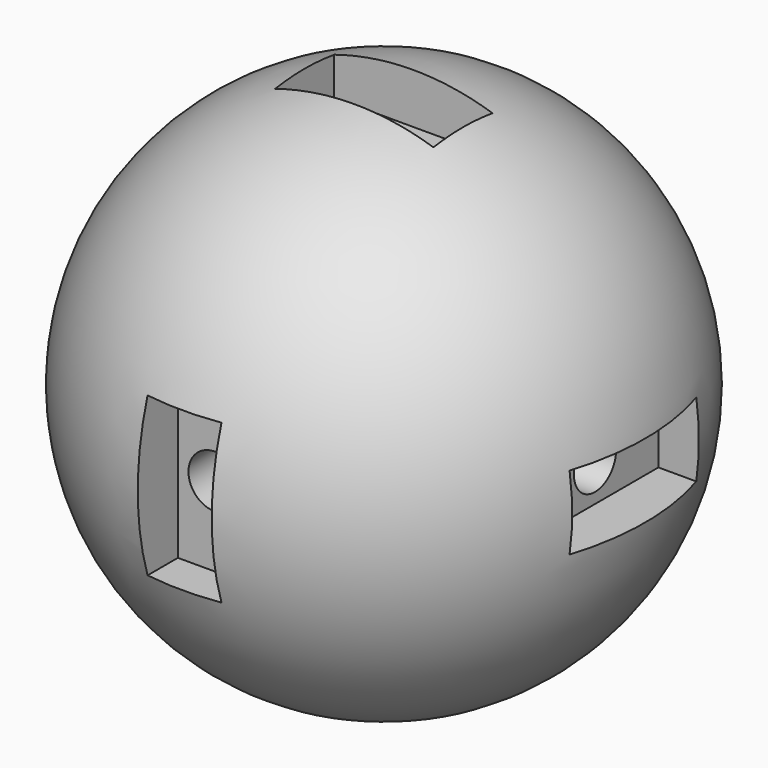
from build123d import *

# Parameters (mm, degrees)
F3_W      = 7
F3_H      = 15
F4_DEPTH  = 5
F5_R      = 2.5
F6_DEPTH  = 45.001
F8_W      = 15
F8_H      = 7
F9_DEPTH  = 5
F10_R     = 2.5
F11_DEPTH = 44.754787589
F13_W     = 15
F13_H     = 7
F14_DEPTH = 5
F15_R     = 2.5
F16_DEPTH = 44.754787589


# Not quite as in the source:
# - a pattern or mirror of a feature is missing from the dataset's text; its kind, count and spacing are read off the source's solid


with BuildPart() as f1:
    # F0 (on Front) → F1 (revolve)
    with BuildSketch(Plane.XZ):
        with BuildLine():
            Line((0, -25), (0, 25))
            ThreePointArc((0, 25), (-25, 0), (0, -25))
        make_face()
    revolve(axis=Axis((0, 0, 0), (0, 0, -1)))

    # F3 (on offset) → F4 (cut)
    with BuildSketch(Plane.XZ.offset(25)):
        Rectangle(F3_W, F3_H)
    f4 = extrude(amount=-F4_DEPTH, mode=Mode.SUBTRACT)

    # F4_copies: F4 across plane
    add(f4.mirror(Plane.ZX), mode=Mode.SUBTRACT)

    # F5 (on face) → F6 (cut, through all)
    with BuildSketch(Plane.XZ.offset(20)):
        Circle(F5_R)
    extrude(amount=-F6_DEPTH, mode=Mode.SUBTRACT)

    # F8 (on offset) → F9 (cut)
    with BuildSketch(Plane.XY.offset(25)):
        Rectangle(F8_W, F8_H)
    f9 = extrude(amount=-F9_DEPTH, mode=Mode.SUBTRACT)

    # F9_copies: F9 across plane
    add(f9.mirror(Plane(origin=(0, 0, 0), x_dir=(-1, 0, 0), z_dir=(0, 0, -1))), mode=Mode.SUBTRACT)

    # F10 (on face) → F11 (cut, through all)
    with BuildSketch(Plane.XY.offset(20)):
        Circle(F10_R)
    extrude(amount=-F11_DEPTH, mode=Mode.SUBTRACT)

    # F13 (on offset) → F14 (cut)
    with BuildSketch(Plane.YZ.offset(25)):
        Rectangle(F13_W, F13_H)
    f14 = extrude(amount=-F14_DEPTH, mode=Mode.SUBTRACT)

    # F14_copies: F14 across plane
    add(f14.mirror(Plane(origin=(0, 0, 0), x_dir=(0, 0, -1), z_dir=(-1, 0, 0))), mode=Mode.SUBTRACT)

    # F15 (on face) → F16 (cut, through all)
    with BuildSketch(Plane.YZ.offset(20)):
        Circle(F15_R)
    extrude(amount=-F16_DEPTH, mode=Mode.SUBTRACT)


solid = f1.part
